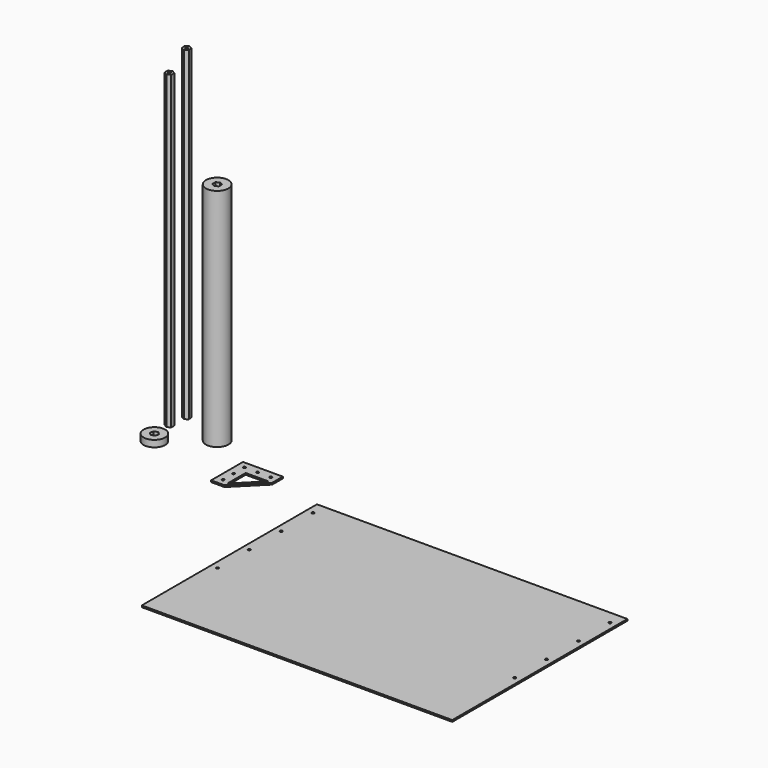
from build123d import *

# Parameters (mm, degrees)
F0_R      = 2.5527
F1_DEPTH  = 622.3
F2_R      = 21.59
F3_DEPTH  = 431.8
F4_W      = 594.36
F4_H      = 419.1
F4_R      = 2.413
F5_DEPTH  = 3.175
F6_R      = 2.5527
F7_DEPTH  = 594.36
F8_R      = 20.6375
F9_DEPTH  = 12.7
F10_R     = 2.38125
F11_DEPTH = 3.175


# Not quite as in the source:
# - a length typed as a fraction of an inch, garbled in the dataset ("3 / 203.2 mm" for 3/8 in), is restored


with BuildPart() as f1:
    # F0 (on Top) → F1 (new body)
    with BuildSketch(Plane.XY):
        Polygon((-58.7014258881, 57.6698564189), (-52.7280128831, 61.9221111625), (-53.423867012, 69.221365944), (-60.0931341459, 72.2683659818), (-66.0665471509, 68.0161112382), (-65.370693022, 60.7168564567), align=None)
        with Locations((-59.397280017, 64.9691112003)):
            Circle(F0_R, mode=Mode.SUBTRACT)
    extrude(amount=F1_DEPTH)


with BuildPart() as f3:
    # F2 (on Top) → F3 (new body)
    with BuildSketch(Plane.XY):
        with Locations((23.0263769627, 34.9923484027)):
            Circle(F2_R)
        Polygon((29.2969861089, 38.7927160519), (29.4528964637, 31.4620254095), (23.1822873174, 27.6616577603), (16.7557678164, 31.1919807536), (16.5998574617, 38.522671396), (22.8704666079, 42.3230390451), align=None, mode=Mode.SUBTRACT)
    extrude(amount=F3_DEPTH)


with BuildPart() as f5:
    # F4 (on Top) → F5 (new body)
    with BuildSketch(Plane.XY):
        with Locations((569.643709116, -247.6076417923)):
            Rectangle(F4_W, F4_H)
        with Locations((285.163709116, -292.0576417923)):
            Circle(F4_R, mode=Mode.SUBTRACT)
        with Locations((854.123709116, -292.0576417923)):
            Circle(F4_R, mode=Mode.SUBTRACT)
        with Locations((285.163709116, -215.8576417923)):
            Circle(F4_R, mode=Mode.SUBTRACT)
        with Locations((285.163709116, -139.6576417923)):
            Circle(F4_R, mode=Mode.SUBTRACT)
        with Locations((285.163709116, -63.4576417923)):
            Circle(F4_R, mode=Mode.SUBTRACT)
        with Locations((854.123709116, -215.8576417923)):
            Circle(F4_R, mode=Mode.SUBTRACT)
        with Locations((854.123709116, -139.6576417923)):
            Circle(F4_R, mode=Mode.SUBTRACT)
        with Locations((854.123709116, -63.4576417923)):
            Circle(F4_R, mode=Mode.SUBTRACT)
    extrude(amount=F5_DEPTH)


with BuildPart() as f7:
    # F6 (on Top) → F7 (new body)
    with BuildSketch(Plane.XY):
        Polygon((-63.2050597455, 21.2249688073), (-56.8484997376, 24.8797572006), (-56.8353593278, 32.2120938447), (-63.1787789258, 35.8896420955), (-69.5353389336, 32.2348537022), (-69.5484793434, 24.9025170581), align=None)
        with Locations((-63.1919193356, 28.5573054514)):
            Circle(F6_R, mode=Mode.SUBTRACT)
    extrude(amount=F7_DEPTH)


with BuildPart() as f9:
    # F8 (on Top) → F9 (new body)
    with BuildSketch(Plane.XY):
        with Locations((-48.9900968969, -25.1767020673)):
            Circle(F8_R)
        Polygon((-41.9728598269, -23.0502690828), (-43.6399333779, -30.190591142), (-50.6571704479, -32.3170241264), (-56.0073339668, -27.3031350517), (-54.3402604158, -20.1628129925), (-47.3230233459, -18.0363800081), align=None, mode=Mode.SUBTRACT)
    extrude(amount=F9_DEPTH)


with BuildPart() as f11:
    # F10 (on Top) → F11 (new body)
    with BuildSketch(Plane.XY):
        Polygon((100.4340276122, 0), (100.4340276122, -76.2), (125.8340276122, -76.2), (176.6340276122, -25.4), (176.6340276122, 0), align=None)
        with Locations((113.1340276122, -63.5)):
            Circle(F10_R, mode=Mode.SUBTRACT)
        Polygon((125.8340276122, -25.4), (169.4498227154, -25.4), (125.8340276122, -69.0157951031), align=None, mode=Mode.SUBTRACT)
        with Locations((113.1340276122, -38.1)):
            Circle(F10_R, mode=Mode.SUBTRACT)
        with Locations((113.1340276122, -12.7)):
            Circle(F10_R, mode=Mode.SUBTRACT)
        with Locations((138.5340276122, -12.7)):
            Circle(F10_R, mode=Mode.SUBTRACT)
        with Locations((163.9340276122, -12.7)):
            Circle(F10_R, mode=Mode.SUBTRACT)
    extrude(amount=F11_DEPTH)


solid = Compound([f1.part, f3.part, f5.part, f7.part, f9.part, f11.part])
